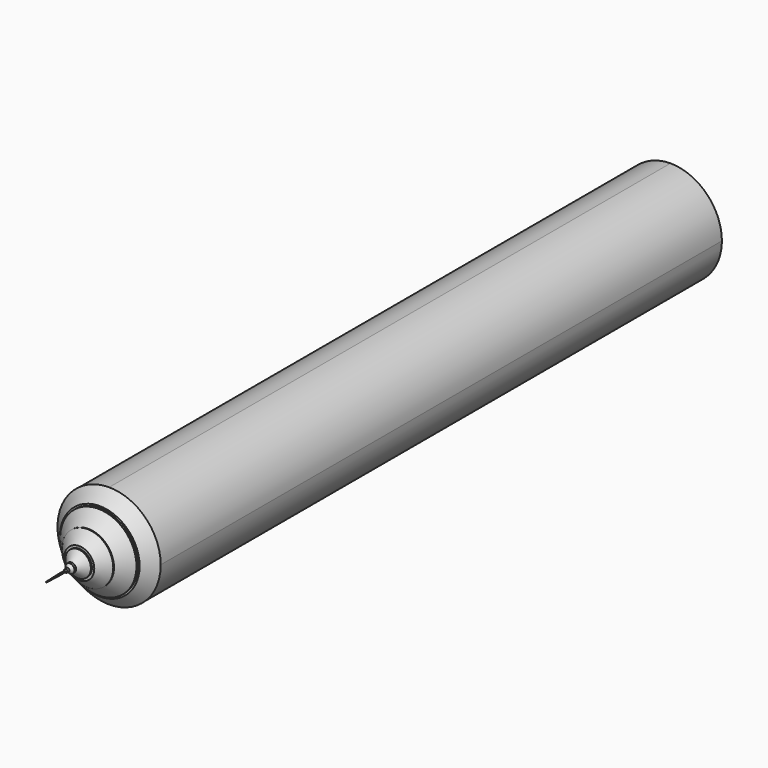
from build123d import *

# Parameters (mm, degrees)
F0_R         = 116.8568622496
F0_R_2       = 82.6855352884
F1_DEPTH     = 25.4
F0_R_3       = 55.5609891669
F3_DEPTH     = 57.15
F0_R_4       = 27.6263375127
F5_DEPTH     = 81.026
F6_SIZE      = 22.86
F0_R_5       = 9.8587759807
F7_DEPTH     = 109.22
F0_R_6       = 3.9101861175
F9_DEPTH     = 113.792
F11_R        = 3.8737007973
F12_DEPTH    = 119.888
F13_SIZE     = 2.54
F14_W        = 222.5426733494
F14_H        = 1520.0280845165
F15_DEPTH    = 111.76
F16_T1_DEPTH = 2081.1154585477
F17_W        = 3.0455216765
F17_H        = 18.2308778167
F18_DEPTH    = 0.8952179924


# Not quite as in the source:
# - a fillet or chamfer that OpenCascade refuses, or shapes differently, is made with other operations: its cross-section is extruded or revolved along the edge and cut away or added


with BuildPart() as f1:
    # F0 (on Front) → F1 (new body)
    with BuildSketch(Plane.XZ):
        Circle(F0_R)
        Circle(F0_R_2, mode=Mode.SUBTRACT)
    extrude(amount=F1_DEPTH)

    # F2: chamfer of 30.48 on 1 edges, made by hand

    # F2_s1 → F2_t2 (revolve, cut)
    with BuildSketch(Plane.XY):
        Polygon((116.8568622496, 5.08), (86.3768622496, -25.4), (116.8568622496, -25.4), align=None)
    revolve(axis=Axis((0, -25.4, 0), (0, -1, 0)), mode=Mode.SUBTRACT)

    # F0 (on Front) → F3 (join)
    with BuildSketch(Plane.XZ):
        Circle(F0_R_2)
        Circle(F0_R_3, mode=Mode.SUBTRACT)
    extrude(amount=F3_DEPTH)

    # F4: chamfer of 27.94 on 1 edges, made by hand

    # F4_s1 → F4_t2 (revolve, cut)
    with BuildSketch(Plane.XY):
        Polygon((82.6855352884, -29.21), (54.7455352884, -57.15), (82.6855352884, -57.15), align=None)
    revolve(axis=Axis((0, -57.15, 0), (0, -1, 0)), mode=Mode.SUBTRACT)

    # F0 (on Front) → F5 (join)
    with BuildSketch(Plane.XZ):
        Circle(F0_R_3)
        Circle(F0_R_4, mode=Mode.SUBTRACT)
    extrude(amount=F5_DEPTH)

    # F6
    f6_edges = [f1.edges().sort_by_distance(p)[0] for p in [
        (-55.560989, -81.026, 0),
    ]]
    chamfer(f6_edges, length=F6_SIZE)

    # F0 (on Front) → F7 (join)
    with BuildSketch(Plane.XZ):
        Circle(F0_R_4)
        Circle(F0_R_5, mode=Mode.SUBTRACT)
    extrude(amount=F7_DEPTH)

    # F8: chamfer of 25.4 on 1 edges, made by hand

    # F8_s1 → F8_t2 (revolve, cut)
    with BuildSketch(Plane.XY):
        Polygon((27.6263375127, -83.82), (2.2263375127, -109.22), (27.6263375127, -109.22), align=None)
    revolve(axis=Axis((0, -109.22, 0), (0, -1, 0)), mode=Mode.SUBTRACT)

    # F0 (on Front) → F9 (join)
    with BuildSketch(Plane.XZ):
        Circle(F0_R_5)
        Circle(F0_R_6, mode=Mode.SUBTRACT)
    extrude(amount=F9_DEPTH)

    # F10: chamfer of 7.62 on 1 edges, made by hand

    # F10_s1 → F10_t2 (revolve, cut)
    with BuildSketch(Plane.XY):
        Polygon((9.8587759807, -106.172), (2.2387759807, -113.792), (9.8587759807, -113.792), align=None)
    revolve(axis=Axis((0, -113.792, 0), (0, -1, 0)), mode=Mode.SUBTRACT)


with BuildPart() as f12:
    # F11 (on face) → F12 (new body)
    with BuildSketch(Plane.XZ):
        Circle(F11_R)
    extrude(amount=F12_DEPTH)

    # F13
    f13_edges = [f12.edges().sort_by_distance(p)[0] for p in [
        (-3.873701, -119.888, 0),
    ]]
    chamfer(f13_edges, length=F13_SIZE)


with BuildPart() as f15:
    # F14 (on Top) → F15 (new body, symmetric)
    with BuildSketch(Plane.XY):
        with Locations((0.1479163766, 760.0140422583)):
            Rectangle(F14_W, F14_H)
    extrude(amount=F15_DEPTH, both=True)

    # F16: fillet of radius 112.2174748062 on 4 edges, made by hand

    # F16_s2 → F16_t1 (cut)
    with BuildSketch(Plane.XZ.offset(-1800.5717715321)):
        with BuildLine():
            ThreePointArc((-111.1234202981, 0.4574748062), (-78.255682895, -78.8922625969), (1.0940545081, -111.76))
            Line((1.0940545081, -111.76), (-111.1234202981, -111.76))
            Line((-111.1234202981, -111.76), (-111.1234202981, 0.4574748062))
        make_face()
        with BuildLine():
            ThreePointArc((111.4192530513, 0.4574748062), (78.5515156482, -78.8922625969), (-0.7982217549, -111.76))
            Line((-0.7982217549, -111.76), (111.4192530513, -111.76))
            Line((111.4192530513, -111.76), (111.4192530513, 0.4574748062))
        make_face()
        with BuildLine():
            ThreePointArc((111.4192530513, -0.4574748062), (78.5515156482, 78.8922625969), (-0.7982217549, 111.76))
            Line((-0.7982217549, 111.76), (111.4192530513, 111.76))
            Line((111.4192530513, 111.76), (111.4192530513, -0.4574748062))
        make_face()
        with BuildLine():
            ThreePointArc((-111.1234202981, -0.4574748062), (-78.255682895, 78.8922625969), (1.0940545081, 111.76))
            Line((1.0940545081, 111.76), (-111.1234202981, 111.76))
            Line((-111.1234202981, 111.76), (-111.1234202981, -0.4574748062))
        make_face()
    extrude(amount=F16_T1_DEPTH, mode=Mode.SUBTRACT)


with BuildPart() as f18:
    # F17 (on Top) → F18 (new body, symmetric)
    with BuildSketch(Plane.XY):
        with Locations((-0.0058300793, -129.0746219456)):
            Rectangle(F17_W, F17_H)
        Polygon((1.516930759, -138.190060854), (-1.5285909176, -138.190060854), (0, -170.647457242), align=None)
    extrude(amount=F18_DEPTH, both=True)


solid = Compound([f1.part, f12.part, f15.part, f18.part])
